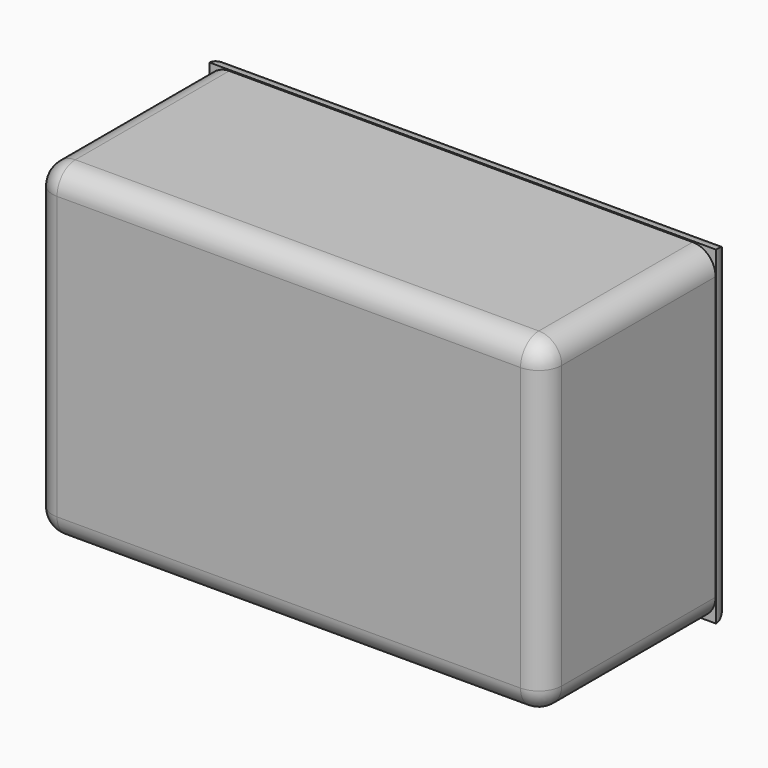
from build123d import *

# Parameters (mm, degrees)
F0_W        = 101.22
F0_H        = 61.63
F1_DEPTH    = 5
F2_R        = 4.99999
F3_W        = 101.22
F3_H        = 61.63
F5_DEPTH    = 42
F6_W        = 4.8751346767
F6_H        = 71.9082504511
F7_DEPTH    = 110.6
F8_T1_DEPTH = 96.9004535608
F8_T3_DEPTH = 135.5922031097


# Not quite as in the source:
# - a fillet or chamfer that OpenCascade refuses, or shapes differently, is made with other operations: its cross-section is extruded or revolved along the edge and cut away or added
# - a fillet or chamfer is up to 0.001 mm smaller than in the source, because OpenCascade refuses the exact size


with BuildPart() as f1:
    # F0 (on Front) → F1 (new body)
    with BuildSketch(Plane.XZ):
        with BuildLine():
            Line((0, 66.63), (-101.22, 66.63))
            ThreePointArc((-101.22, 66.63), (-104.7555339059, 65.1655339059), (-106.22, 61.63))
            Line((-106.22, 61.63), (-106.22, 0))
            ThreePointArc((-106.22, 0), (-104.7555339059, -3.5355339059), (-101.22, -5))
            Line((-101.22, -5), (0, -5))
            ThreePointArc((0, -5), (3.5355339059, -3.5355339059), (5, 0))
            Line((5, 0), (5, 61.63))
            ThreePointArc((5, 61.63), (3.5355339059, 65.1655339059), (0, 66.63))
        make_face()
        with Locations((-50.61, 30.815)):
            Rectangle(F0_W, F0_H, mode=Mode.SUBTRACT)
        with Locations((-50.61, 30.815)):
            Rectangle(F0_W, F0_H)
    extrude(amount=F1_DEPTH)

    # F2 (radius 5 in the source; OpenCascade refuses exactly that, so slightly less here)
    f2_edges = [f1.edges().sort_by_distance(p)[0] for p in [
        (-50.61, -5, -5),
    ]]
    fillet(f2_edges, radius=F2_R)

    # F3 (on face) → F5 (join)
    with BuildSketch(Plane(origin=(0, 0, 0), x_dir=(-1, 0, 0), z_dir=(0, 1, 0))):
        with BuildLine():
            Line((101.22, 66.63), (0, 66.63))
            ThreePointArc((0, 66.63), (-3.5355339059, 65.1655339059), (-5, 61.63))
            Line((-5, 61.63), (-5, 0))
            ThreePointArc((-5, 0), (-3.5355339059, -3.5355339059), (0, -5))
            Line((0, -5), (101.22, -5))
            ThreePointArc((101.22, -5), (104.7555339059, -3.5355339059), (106.22, 0))
            Line((106.22, 0), (106.22, 61.63))
            ThreePointArc((106.22, 61.63), (104.7555339059, 65.1655339059), (101.22, 66.63))
        make_face()
        with Locations((50.61, 30.815)):
            Rectangle(F3_W, F3_H, mode=Mode.SUBTRACT)
    extrude(amount=F5_DEPTH)


with BuildPart() as f7:
    # F6 (on face) → F7 (new body)
    with BuildSketch(Plane.YZ.offset(5)):
        with Locations((44.5501934737, 30.8286100626)):
            Rectangle(F6_W, F6_H)
    extrude(amount=-F7_DEPTH)

    # F8: fillet of radius 5 on 4 edges, made by hand

    # F8_s2 → F8_t1 (cut)
    with BuildSketch(Plane.XY.offset(-17.6216167178)):
        with BuildLine():
            ThreePointArc((0.0015593781, 46.987760812), (3.4926676107, 45.5671690464), (5, 42.1126261353))
            Line((5, 42.1126261353), (5, 46.987760812))
            Line((5, 46.987760812), (0.0015593781, 46.987760812))
        make_face()
        with BuildLine():
            ThreePointArc((-100.6015593781, 46.987760812), (-104.0926676107, 45.5671690464), (-105.6, 42.1126261353))
            Line((-105.6, 42.1126261353), (-105.6, 46.987760812))
            Line((-105.6, 46.987760812), (-100.6015593781, 46.987760812))
        make_face()
    extrude(amount=F8_T1_DEPTH, mode=Mode.SUBTRACT)

    # F8_s4 → F8_t3 (cut)
    with BuildSketch(Plane.YZ.offset(-118.0961015548)):
        with BuildLine():
            ThreePointArc((42.1126261353, 66.7827352881), (45.5671690464, 65.2754028988), (46.987760812, 61.7842946662))
            Line((46.987760812, 61.7842946662), (46.987760812, 66.7827352881))
            Line((46.987760812, 66.7827352881), (42.1126261353, 66.7827352881))
        make_face()
        with BuildLine():
            ThreePointArc((42.1126261353, -5.1255151629), (45.5671690464, -3.6181827736), (46.987760812, -0.127074541))
            Line((46.987760812, -0.127074541), (46.987760812, -5.1255151629))
            Line((46.987760812, -5.1255151629), (42.1126261353, -5.1255151629))
        make_face()
    extrude(amount=F8_T3_DEPTH, mode=Mode.SUBTRACT)


solid = Compound([f1.part, f7.part])
